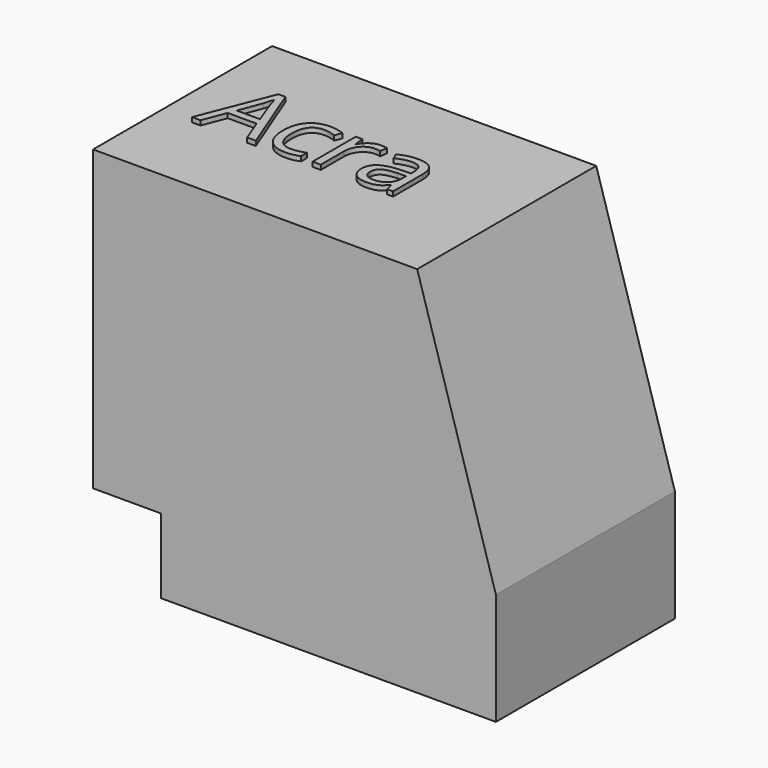
from build123d import *

# Parameters (mm, degrees)
F0_W         = 2160
F0_H         = 1200
F1_DEPTH     = 2000
F3_DEPTH     = 1200.001
F4_W         = 365
F4_H         = 400
F5_DEPTH     = 1200.001
F6_TEXT_SIZE = 540.9321851201
F7_DEPTH     = 25


# Not quite as in the source:
# - Text() gives the source's letters only with a copy of the font that has no kerning and outlines rounded to 1/6400 em; it was checked with that copy


with BuildPart() as f1:
    # F0 (on Top) → F1 (new body)
    with BuildSketch(Plane.XY):
        with Locations((1080, -600)):
            Rectangle(F0_W, F0_H)
    extrude(amount=F1_DEPTH)

    # F2 (on face) → F3 (cut, through all)
    with BuildSketch(Plane.XZ.offset(1200)):
        Polygon((1738.0541563034, 2000), (2160, 600), (2160, 2000), align=None)
    extrude(amount=-F3_DEPTH, mode=Mode.SUBTRACT)

    # F4 (on face) → F5 (cut, through all)
    with BuildSketch(Plane.XZ.offset(1200)):
        with Locations((182.5, 200)):
            Rectangle(F4_W, F4_H)
    extrude(amount=-F5_DEPTH, mode=Mode.SUBTRACT)

    # F6 (on face) → F7 (join)
    with BuildSketch(Plane.XY.offset(2000)):
        with Locations((170.5310642719, -749.7934699059)):
            Text('Acra', F6_TEXT_SIZE, font='Open Sans', text_align=(TextAlign.LEFT, TextAlign.BOTTOM))
    extrude(amount=F7_DEPTH)


solid = f1.part
